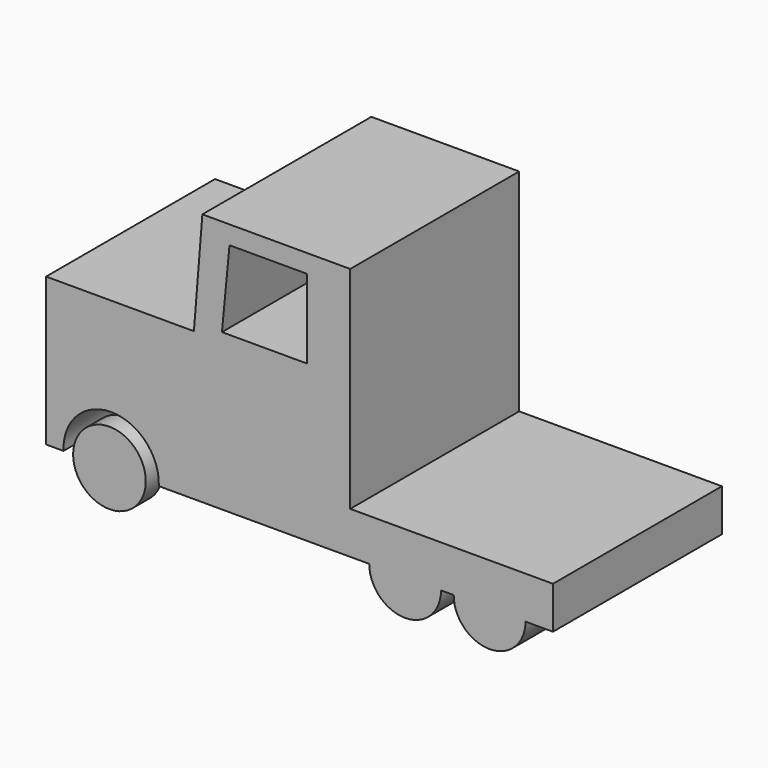
from build123d import *

# Parameters (mm, degrees)
F1_DEPTH = 31.75
F2_DEPTH = 31.75
F3_DEPTH = 25.4
F4_DEPTH = 25.4
F5_DEPTH = 15.875
F7_DEPTH = 25.4


with BuildPart() as f1:
    # F0 (on Front) → F1 (new body, symmetric)
    with BuildSketch(Plane.XZ):
        with BuildLine():
            Line((-50.6557935558, 27.335102257), (-50.6557935558, -17.114897743))
            Line((-50.6557935558, -17.114897743), (-45.4152002931, -17.114897743))
            ThreePointArc((-45.4152002931, -17.114897743), (-31.0896001756, -2.1471956478), (-16.7640000582, -17.114897743))
            Line((-16.7640000582, -17.114897743), (46.4992064442, -17.114897743))
            ThreePointArc((46.4992064442, -17.114897743), (57.2942064442, -6.319897743), (68.0892064442, -17.114897743))
            Line((68.0892064442, -17.114897743), (71.8992064442, -17.114897743))
            ThreePointArc((71.8992064442, -17.114897743), (82.6942064442, -6.319897743), (93.4892064442, -17.114897743))
            Line((93.4892064442, -17.114897743), (101.7442064442, -17.114897743))
            Line((101.7442064442, -17.114897743), (101.7442064442, -4.414897743))
            Line((101.7442064442, -4.414897743), (69.7991997004, -4.414897743))
            Line((69.7991997004, -4.414897743), (65.5320063233, -4.414897743))
            Line((65.5320063233, -4.414897743), (40.7842064442, -4.414897743))
            Line((40.7842064442, -4.414897743), (40.7842064442, 59.085102257))
            Line((40.7842064442, 59.085102257), (-3.6657935558, 59.085102257))
            Line((-3.6657935558, 59.085102257), (-6.2057935558, 27.335102257))
            Line((-6.2057935558, 27.335102257), (-50.6557935558, 27.335102257))
        make_face()
        Polygon((27.7291558257, 29.8314392567), (2.2207412403, 29.8314392567), (4.4933222234, 53.5672903061), (27.7241561562, 53.5672903061), align=None, mode=Mode.SUBTRACT)
        with BuildLine():
            ThreePointArc((68.0892064442, -17.114897743), (57.2942064442, -6.319897743), (46.4992064442, -17.114897743))
            Line((46.4992064442, -17.114897743), (68.0892064442, -17.114897743))
        make_face()
        with BuildLine():
            ThreePointArc((93.4892064442, -17.114897743), (82.6942064442, -6.319897743), (71.8992064442, -17.114897743))
            Line((71.8992064442, -17.114897743), (93.4892064442, -17.114897743))
        make_face()
    extrude(amount=F1_DEPTH, both=True)

    # F0 (on Front) → F2, piece 2 (join, symmetric)
    with BuildSketch(Plane.XZ):
        with BuildLine():
            Line((68.0892064442, -17.114897743), (46.4992064442, -17.114897743))
            ThreePointArc((46.4992064442, -17.114897743), (57.2942064442, -27.909897743), (68.0892064442, -17.114897743))
        make_face()
        with BuildLine():
            Line((93.4892064442, -17.114897743), (71.8992064442, -17.114897743))
            ThreePointArc((71.8992064442, -17.114897743), (82.6942064442, -27.909897743), (93.4892064442, -17.114897743))
        make_face()
    extrude(amount=F2_DEPTH, both=True)

    # F0 (on Front) → F5 (cut, symmetric)
    with BuildSketch(Plane.XZ):
        with BuildLine():
            Line((93.4892064442, -17.114897743), (71.8992064442, -17.114897743))
            ThreePointArc((71.8992064442, -17.114897743), (82.6942064442, -27.909897743), (93.4892064442, -17.114897743))
        make_face()
        with BuildLine():
            Line((68.0892064442, -17.114897743), (46.4992064442, -17.114897743))
            ThreePointArc((46.4992064442, -17.114897743), (57.2942064442, -27.909897743), (68.0892064442, -17.114897743))
        make_face()
    extrude(amount=F5_DEPTH, both=True, mode=Mode.SUBTRACT)

    # F6 (on face) → F7 (cut)
    with BuildSketch(Plane(origin=(-8.3392306601, 0, 0.6671384528), x_dir=(0, -1, 0), z_dir=(-0.9968152785, 0, 0.0797452223))):
        Polygon((26.67, 53.5246031417), (-26.6048397136, 53.5246031417), (-26.67, 31.8331651835), (26.67, 31.8331651835), align=None)
    extrude(amount=F7_DEPTH, mode=Mode.SUBTRACT)


with BuildPart() as f2:
    # F0 (on Front) → F2 (new body, symmetric)
    with BuildSketch(Plane.XZ):
        with BuildLine():
            ThreePointArc((-20.6837935558, -17.114897743), (-31.6057935558, -6.192897743), (-42.5277935558, -17.114897743))
            Line((-42.5277935558, -17.114897743), (-20.6837935558, -17.114897743))
        make_face()
        with BuildLine():
            Line((-20.6837935558, -17.114897743), (-42.5277935558, -17.114897743))
            ThreePointArc((-42.5277935558, -17.114897743), (-31.6057935558, -28.036897743), (-20.6837935558, -17.114897743))
        make_face()
    extrude(amount=F2_DEPTH, both=True)

    # F0 (on Front) → F3 (cut, symmetric)
    with BuildSketch(Plane.XZ):
        with BuildLine():
            Line((-20.6837935558, -17.114897743), (-42.5277935558, -17.114897743))
            ThreePointArc((-42.5277935558, -17.114897743), (-31.6057935558, -28.036897743), (-20.6837935558, -17.114897743))
        make_face()
    extrude(amount=F3_DEPTH, both=True, mode=Mode.SUBTRACT)

    # F4 (cut): a face of the model
    f4_faces = [f2.faces().sort_by_distance(p)[0] for p in [
        (-31.6057935558, 0, -17.114897743),
    ]]
    extrude(f4_faces, amount=-F4_DEPTH, mode=Mode.SUBTRACT)


solid = Compound([f1.part, f2.part])
